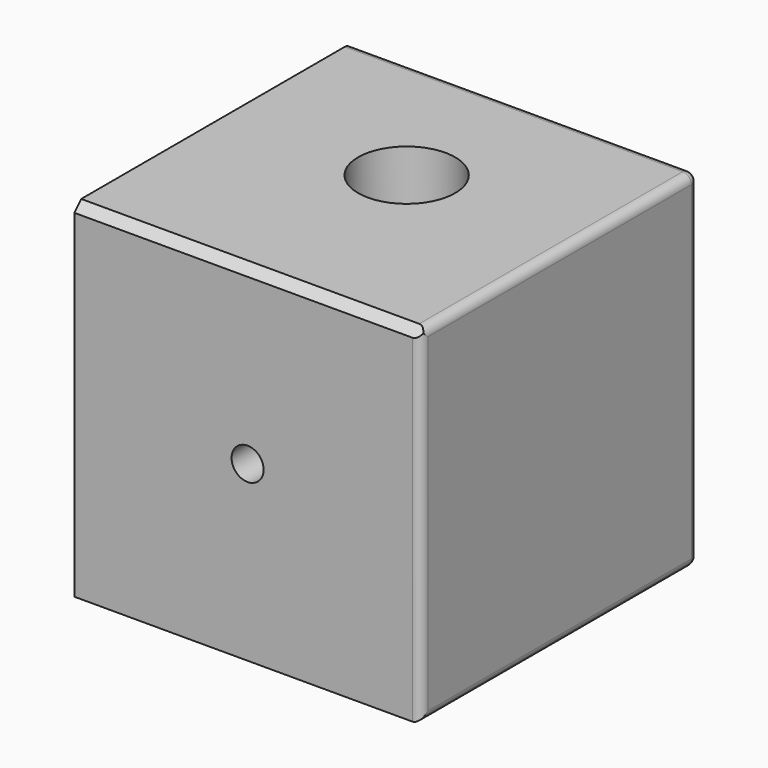
from build123d import *

# Parameters (mm, degrees)
F1_W      = 200
F1_H      = 200
F2_DEPTH  = 100
F4_D      = 18.5
F4_DEPTH  = 22.5
F4_TIP    = 5.557960726
F5_SIZE   = 5
F6_R      = 5
F8_R      = 4.99999
F10_D     = 56
F10_DEPTH = 72
F10_TIP   = 16.8240973328


# Not quite as in the source:
# - a fillet or chamfer is up to 0.001 mm smaller than in the source, because OpenCascade refuses the exact size
# - a feature of the source that left no trace in its solid (it failed there, or was rolled back) is left out


with BuildPart() as f2:
    # F1 (on Front) → F2 (new body, symmetric)
    with BuildSketch(Plane.XZ):
        Rectangle(F1_W, F1_H)
    extrude(amount=F2_DEPTH, both=True)

    # F4
    with Locations(Plane.XZ.offset(100)):
        with Locations((0, 0)):
            Hole(F4_D / 2, depth=F4_DEPTH)
            with Locations((0, 0, -(F4_DEPTH + F4_TIP / 2))):  # 118° drill point
                Cone(0, F4_D / 2, F4_TIP, mode=Mode.SUBTRACT)

    # F5
    f5_edges = [f2.edges().sort_by_distance(p)[0] for p in [
        (0, -100, 100),
    ]]
    chamfer(f5_edges, length=F5_SIZE)

    # F6
    f6_edges = [f2.edges().sort_by_distance(p)[0] for p in [
        (100, 2.5, 100),
    ]]
    fillet(f6_edges, radius=F6_R)

    # F8 (radius 5 in the source; OpenCascade refuses exactly that, so slightly less here)
    f8_edges = [f2.edges().sort_by_distance(p)[0] for p in [
        (0, 100, -100),
        (-2.5, 100, 100),
        (98.535534, 100, 98.535534),
        (100, 100, -2.5),
        (100, -100, -2.5),
        (100, 0, -100),
    ]]
    fillet(f8_edges, radius=F8_R)

    # F10
    with Locations(Plane.XY.offset(100)):
        with Locations((0, 14.7048085928)):
            Hole(F10_D / 2, depth=F10_DEPTH)
            with Locations((0, 0, -(F10_DEPTH + F10_TIP / 2))):  # 118° drill point
                Cone(0, F10_D / 2, F10_TIP, mode=Mode.SUBTRACT)


solid = f2.part
